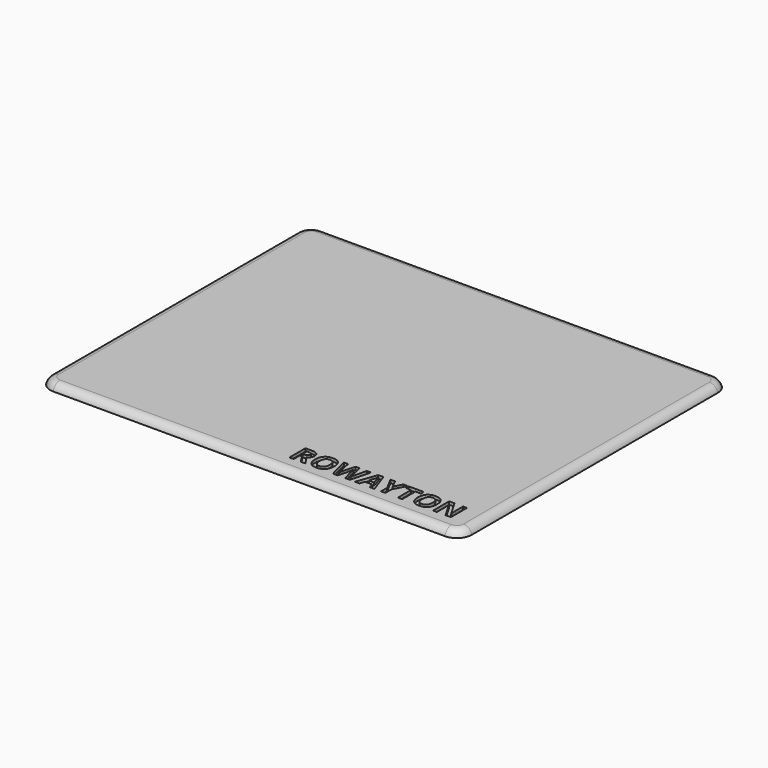
from build123d import *

# Parameters (mm, degrees)
F0_W         = 250
F0_H         = 200
F1_DEPTH     = 4
F2_R         = 8.89
F3_T1_DEPTH  = 182.22
F3_T3_DEPTH  = 232.22
F3_T6_ANGLE  = 90
F3_T8_ANGLE  = 90
F3_T10_ANGLE = 90
F3_T12_ANGLE = 90
F4_TEXT_SIZE = 16.6666666667
F5_DEPTH     = 1.8


# Not quite as in the source:
# - a fillet or chamfer that OpenCascade refuses, or shapes differently, is made with other operations: its cross-section is extruded or revolved along the edge and cut away or added
# - Text() gives the source's letters only with a copy of the font that has no kerning and outlines rounded to 1/6400 em; it was checked with that copy


with BuildPart() as f1:
    # F0 (on Top) → F1 (new body)
    with BuildSketch(Plane.XY):
        Rectangle(F0_W, F0_H)
    extrude(amount=F1_DEPTH)

    # F2
    f2_edges = [f1.edges().sort_by_distance(p)[0] for p in [
        (-125, -100, 2),
        (125, -100, 2),
        (125, 100, 2),
        (-125, 100, 2),
    ]]
    fillet(f2_edges, radius=F2_R)

    # F3: fillet of radius 5.08 on 1 edges, made by hand

    # F3_s2 → F3_t1 (cut)
    with BuildSketch(Plane.XZ.offset(-91.11)):
        with BuildLine():
            ThreePointArc((-120.0361305416, 4), (-123.2236060317, 2.8755530587), (-125, 0))
            Line((-125, 0), (-125, 4))
            Line((-125, 4), (-120.0361305416, 4))
        make_face()
        with BuildLine():
            ThreePointArc((120.0361305416, 4), (123.2236060317, 2.8755530587), (125, 0))
            Line((125, 0), (125, 4))
            Line((125, 4), (120.0361305416, 4))
        make_face()
    extrude(amount=F3_T1_DEPTH, mode=Mode.SUBTRACT)

    # F3_s4 → F3_t3 (cut)
    with BuildSketch(Plane.YZ.offset(-116.11)):
        with BuildLine():
            ThreePointArc((-100, 0), (-98.2236060317, 2.8755530587), (-95.0361305416, 4))
            Line((-95.0361305416, 4), (-100, 4))
            Line((-100, 4), (-100, 0))
        make_face()
        with BuildLine():
            ThreePointArc((95.0361305416, 4), (98.2236060317, 2.8755530587), (100, 0))
            Line((100, 0), (100, 4))
            Line((100, 4), (95.0361305416, 4))
        make_face()
    extrude(amount=F3_T3_DEPTH, mode=Mode.SUBTRACT)

    # F3_s5 → F3_t6 (revolve, cut)
    with BuildSketch(Plane.YZ.offset(-116.11)):
        with BuildLine():
            ThreePointArc((95.0361305416, 4), (98.2236060317, 2.8755530587), (100, 0))
            Line((100, 0), (100, 4))
            Line((100, 4), (95.0361305416, 4))
        make_face()
    revolve(axis=Axis((-116.11, 91.11, 4), (0, 0, 1)), revolution_arc=F3_T6_ANGLE, mode=Mode.SUBTRACT)

    # F3_s7 → F3_t8 (revolve, cut)
    with BuildSketch(Plane.YZ.offset(-116.11)):
        with BuildLine():
            ThreePointArc((-100, 0), (-98.2236060317, 2.8755530587), (-95.0361305416, 4))
            Line((-95.0361305416, 4), (-100, 4))
            Line((-100, 4), (-100, 0))
        make_face()
    revolve(axis=Axis((-116.11, -91.11, 4), (0, 0, -1)), revolution_arc=F3_T8_ANGLE, mode=Mode.SUBTRACT)

    # F3_s9 → F3_t10 (revolve, cut)
    with BuildSketch(Plane.YZ.offset(116.11)):
        with BuildLine():
            ThreePointArc((-100, 0), (-98.2236060317, 2.8755530587), (-95.0361305416, 4))
            Line((-95.0361305416, 4), (-100, 4))
            Line((-100, 4), (-100, 0))
        make_face()
    revolve(axis=Axis((116.11, -91.11, 4), (0, 0, 1)), revolution_arc=F3_T10_ANGLE, mode=Mode.SUBTRACT)

    # F3_s11 → F3_t12 (revolve, cut)
    with BuildSketch(Plane.XZ.offset(-91.11)):
        with BuildLine():
            ThreePointArc((120.0361305416, 4), (123.2236060317, 2.8755530587), (125, 0))
            Line((125, 0), (125, 4))
            Line((125, 4), (120.0361305416, 4))
        make_face()
    revolve(axis=Axis((116.11, 91.11, 4), (0, 0, 1)), revolution_arc=F3_T12_ANGLE, mode=Mode.SUBTRACT)

    # F4 (on face) → F5 (cut)
    with BuildSketch(Plane.XY.offset(4)):
        with Locations((13.9110693708, -89.3684158921)):
            Text('ROWAYTON', F4_TEXT_SIZE, font='Open Sans', font_style=FontStyle.BOLD, text_align=(TextAlign.LEFT, TextAlign.BOTTOM))
    extrude(amount=-F5_DEPTH, mode=Mode.SUBTRACT)


solid = f1.part
